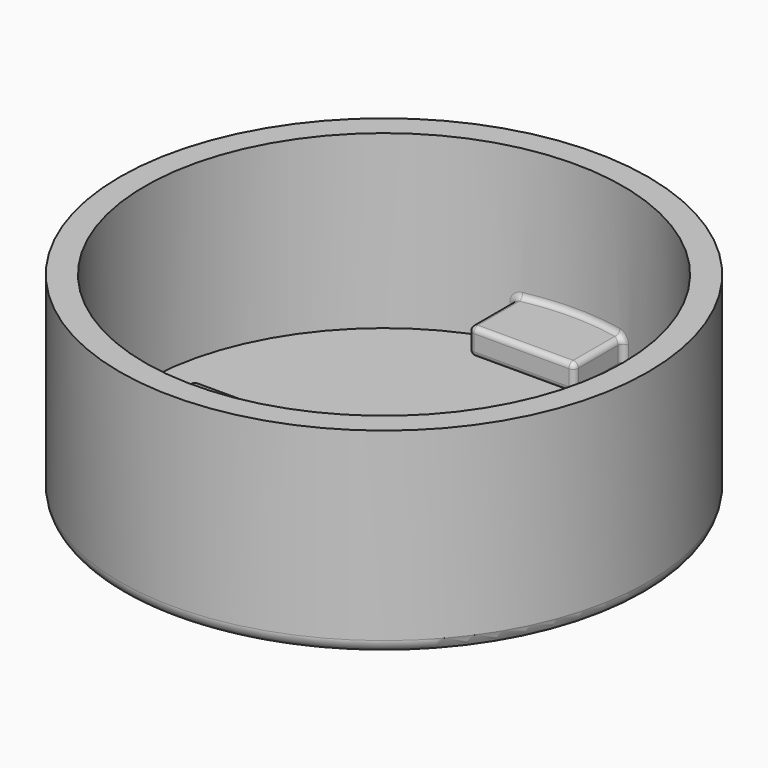
from build123d import *

# Parameters (mm, degrees)
F0_R     = 25.4
F1_DEPTH = 2.54
F2_R     = 25.4
F2_R_2   = 22.987
F3_DEPTH = 16.51
F6_W     = 10.16
F6_H     = 2.54
F8_W     = 10.16
F8_H     = 2.54
F10_R    = 1.27
F11_R    = 0.508


with BuildPart() as f1:
    # F0 (on Top) → F1 (new body)
    with BuildSketch(Plane.XY):
        Circle(F0_R)
    extrude(amount=F1_DEPTH)

    # F2 (on face) → F3 (join)
    with BuildSketch(Plane.XY.offset(2.54)):
        Circle(F2_R)
        Circle(F2_R_2, mode=Mode.SUBTRACT)
    extrude(amount=F3_DEPTH)

    # F6 (on offset) → F7 (join, up to the next surface of F1)
    with BuildSketch(Plane.XZ.offset(16.51)):
        with Locations((0, 13.97)):
            Rectangle(F6_W, F6_H)
    extrude(until=Until.NEXT)

    # F8 (on offset) → F9 (join, up to the next surface of F1)
    with BuildSketch(Plane.XZ.offset(-16.51)):
        with Locations((0, 5.08)):
            Rectangle(F8_W, F8_H)
    extrude(until=Until.NEXT, dir=(0, 1, 0))

    # F10
    f10_edges = [f1.edges().sort_by_distance(p)[0] for p in [
        (-25.4, 0, 0),
    ]]
    fillet(f10_edges, radius=F10_R)

    # F11
    f11_edges = [f1.edges().sort_by_distance(p)[0] for p in [
        (0, -16.51, 15.24),
        (-5.08, -19.464324, 15.24),
        (0, -22.987, 15.24),
        (5.08, -19.464324, 15.24),
        (-5.08, -16.51, 13.97),
        (-5.08, -19.464324, 12.7),
        (-5.08, -22.418648, 13.97),
        (5.08, -16.51, 13.97),
        (5.08, -22.418648, 13.97),
        (5.08, -19.464324, 12.7),
        (0, -16.51, 12.7),
        (25.028026, 0, 0.371974),
        (-25.4, 0, 1.27),
        (-24.13, 0, 0),
        (0, 16.51, 6.35),
        (-5.08, 19.464324, 6.35),
        (0, 22.987, 6.35),
        (5.08, 19.464324, 6.35),
        (5.08, 16.51, 5.08),
        (-5.08, 16.51, 5.08),
        (0, 16.51, 3.81),
        (5.08, 22.418648, 5.08),
        (5.08, 19.464324, 3.81),
        (-5.08, 19.464324, 3.81),
        (-5.08, 22.418648, 5.08),
        (0, -22.987, 12.7),
        (0, 22.987, 3.81),
    ]]
    fillet(f11_edges, radius=F11_R)


solid = f1.part
